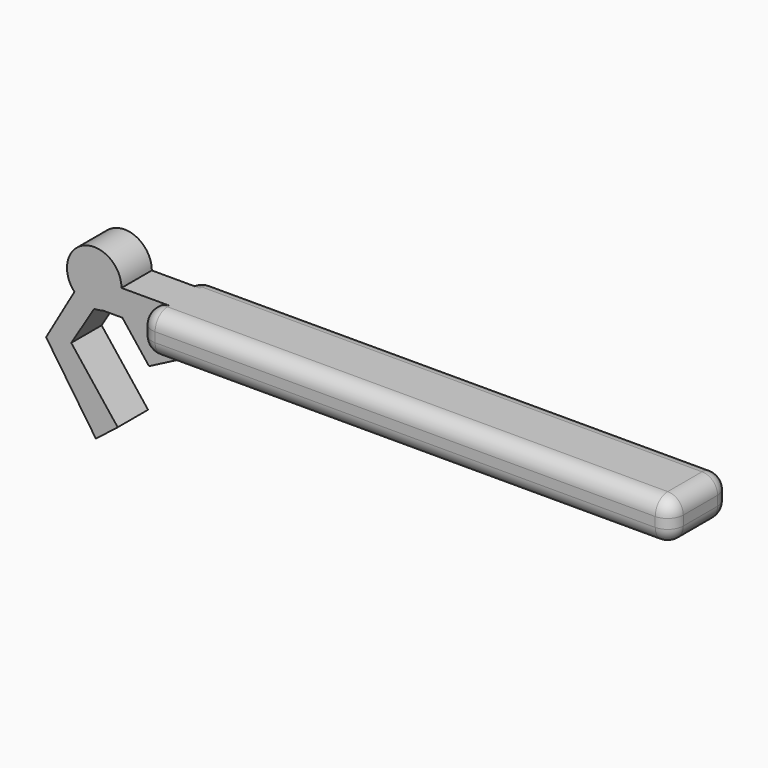
from build123d import *

# Parameters (mm, degrees)
F1_DEPTH = 6.35
F2_W     = 6.35
F2_H     = 4.3350251792
F3_DEPTH = 25.4
F4_DEPTH = 63.5
F5_R     = 2.607278221


# Not quite as in the source:
# - a feature names something its author has since deleted; it is built from what else it names


with BuildPart() as f1:
    # F0 (on Front) → F1 (new body)
    with BuildSketch(Plane.XZ):
        with BuildLine():
            ThreePointArc((38.0586988364, 29.6543792382), (40.3399245407, 31.3092753383), (41.2114633723, 33.9894044175))
            ThreePointArc((41.2114633723, 33.9894044175), (34.9686895654, 38.2226770455), (33.345850058, 30.8565916617))
            ThreePointArc((33.345850058, 30.8565916617), (34.8508967595, 29.8049682674), (36.6488133888, 29.4327141456))
            ThreePointArc((36.6488133888, 29.4327141456), (37.3624884645, 29.4880051728), (38.0586988364, 29.6543792382))
        make_face()
        with BuildLine():
            ThreePointArc((36.6488133888, 29.4327141456), (34.8508967595, 29.8049682674), (33.345850058, 30.8565916617))
            Line((33.345850058, 30.8565916617), (28.5997511098, 22.6370067444))
            Line((28.5997511098, 22.6370067444), (36.9340473419, 10.395447725))
            Line((36.9340473419, 10.395447725), (40.5838886152, 13.2587963652))
            Line((40.5838886152, 13.2587963652), (32.8096505039, 23.1684296974))
            Line((32.8096505039, 23.1684296974), (36.6488133888, 29.4327141456))
        make_face()
        Polygon((56.8539685432, 29.6543792382), (41.3639992476, 29.6543792382), (45.8250723122, 23.9679572756), align=None)
        with BuildLine():
            Line((72.0483290742, 33.9894044175), (41.2114633723, 33.9894044175))
            ThreePointArc((41.2114633723, 33.9894044175), (40.3399245407, 31.3092753383), (38.0586988364, 29.6543792382))
            Line((38.0586988364, 29.6543792382), (41.3639992476, 29.6543792382))
            Line((41.3639992476, 29.6543792382), (56.8539685432, 29.6543792382))
            Line((56.8539685432, 29.6543792382), (72.0483290742, 29.6543792382))
            Line((72.0483290742, 29.6543792382), (72.0483290742, 33.9894044175))
        make_face()
    extrude(amount=F1_DEPTH)

    # F2 (on face) → F3 (join)
    with BuildSketch(Plane.YZ.offset(72.0483290742)):
        Polygon((-6.35, 29.6543792382), (-6.35, 33.9894044175), (-9.3679074198, 33.9894044175), (-9.3679074198, 27.1660927683), (3.0179074198, 27.1660927683), (3.0179074198, 33.9894044175), (0, 33.9894044175), (0, 29.6543792382), align=None)
        with Locations((-3.175, 31.8218918279)):
            Rectangle(F2_W, F2_H)
    extrude(amount=-F3_DEPTH)

    # F4 (add): a face of the model
    f4_faces = [f1.faces().sort_by_distance(p)[0] for p in [
        (72.0483290742, -3.175, 30.5777485929),
    ]]
    extrude(f4_faces, amount=F4_DEPTH)

    # F5
    f5_edges = [f1.edges().sort_by_distance(p)[0] for p in [
        (91.098329, 3.017907, 33.989404),
        (91.098329, 3.017907, 27.166093),
        (91.098329, -9.367907, 27.166093),
        (91.098329, -9.367907, 33.989404),
        (135.548329, -3.175, 33.989404),
        (135.548329, -3.175, 27.166093),
        (135.548329, -9.367907, 30.577749),
        (135.548329, 3.017907, 30.577749),
        (46.648329, 3.017907, 30.577749),
        (46.648329, 1.508954, 33.989404),
        (46.648329, 1.508954, 27.166093),
        (46.648329, -7.858954, 33.989404),
        (46.648329, -7.858954, 27.166093),
        (46.648329, -9.367907, 30.577749),
    ]]
    fillet(f5_edges, radius=F5_R)


solid = f1.part
